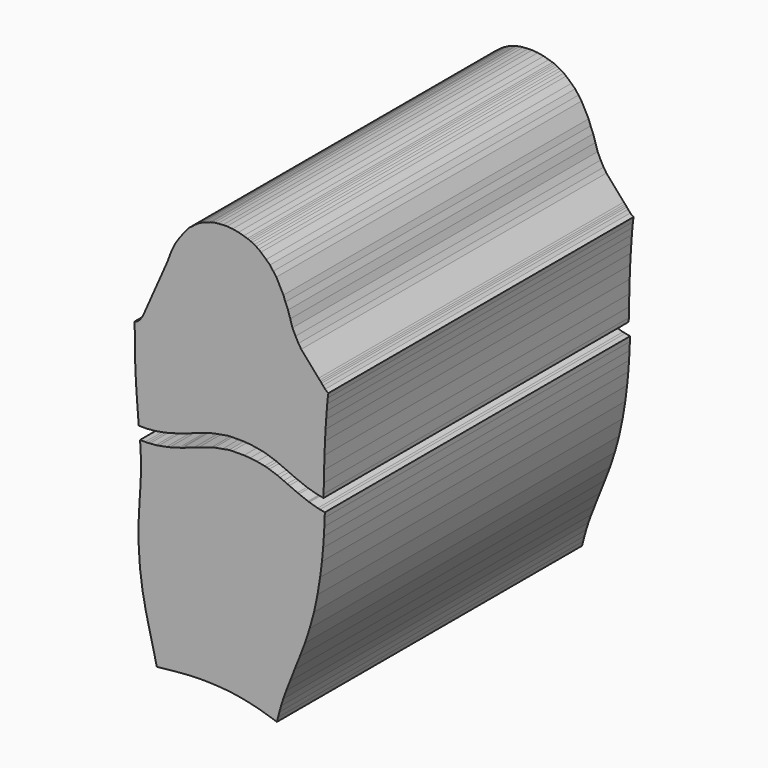
from build123d import *

# Parameters (mm, degrees)
F2_DEPTH = 508


# Not quite as in the source:
# - the program builds the solid bodies; features that only make, move or delete a surface that nothing else refers to are left out


with BuildPart() as f2:
    # F0 (on Front) → F2 (new body)
    with BuildSketch(Plane.XZ):
        Polygon((-99.35524, -267.157394), (-87.704154, -265.912724), (-77.642191, -264.889562), (-67.687226, -263.950115), (-57.626497, -263.202614), (-47.835855, -262.752223), (-37.623644, -262.622648), (-27.549122, -262.832515), (-17.617123, -263.335506), (-7.703785, -264.137581), (1.93555, -265.255393), (11.78373, -266.764753), (21.403733, -268.685028), (30.708282, -270.83535), (39.779716, -273.220339), (47.856634, -275.617817), (54.708213, -277.79442), (60.621898, -279.7178), (62.100178, -273.892381), (63.860292, -267.155842), (66.065188, -259.260817), (68.922512, -250.058256), (72.873976, -239.227413), (78.009644, -226.195026), (84.088358, -210.560021), (90.96442, -193.298534), (97.880029, -175.224811), (104.237719, -155.856182), (109.972263, -134.97015), (114.571321, -113.121317), (118.10686, -91.616372), (120.577504, -72.156973), (122.125705, -55.726912), (123.12777, -41.873435), (123.758995, -30.217446), (124.191324, -19.726469), (124.403661, -13.319637), (118.051474, -12.002012), (114.902297, -11.379006), (103.790009, -8.175114), (102.941473, -7.932579), (102.774185, -7.869009), (101.851989, -7.507658), (90.04621, -2.907224), (87.941009, -2.099751), (77.087624, 2.698767), (74.31532, 3.890768), (69.497222, 5.997663), (64.486402, 8.188801), (61.150429, 9.579169), (50.325408, 13.192707), (47.439086, 14.157448), (44.15215, 14.980091), (33.917572, 16.920968), (24.832063, 18.047035), (16.925466, 18.617653), (1.300727, 18.502788), (-3.02828, 18.408632), (-11.997373, 16.688876), (-22.540419, 14.802432), (-26.847447, 13.566969), (-43.403485, 8.30176), (-49.739938, 6.067019), (-65.069438, 0.721942), (-65.631731, 0.525868), (-66.822744, 0.149595), (-69.900765, -0.691604), (-82.198069, -4.148932), (-86.677218, -5.146552), (-96.860889, -7.030491), (-100.650569, -7.635152), (-108.615022, -8.256464), (-111.81327, -8.50803), (-114.846382, -8.486087), (-121.66787, -8.40389), (-121.242843, -14.793437), (-120.757245, -23.907133), (-120.423058, -34.545006), (-120.480208, -47.140266), (-121.136163, -62.259157), (-122.286607, -80.620535), (-123.449045, -102.956413), (-123.594037, -129.314381), (-121.806265, -157.957926), (-118.219785, -184.666238), (-113.801807, -206.999505), (-109.393073, -225.58084), (-105.540493, -241.278075), (-102.235424, -254.856704), align=None)
    extrude(amount=F2_DEPTH)


with BuildPart() as f2b:
    # F0 (on Front) → F2, piece 2 (new body)
    with BuildSketch(Plane.XZ):
        Polygon((-125.782705, 128.917153), (-129.062374, 127.987089), (-128.75574, 122.909312), (-128.690088, 116.899531), (-128.652305, 109.84454), (-128.59512, 101.393501), (-128.429667, 91.558586), (-128.095552, 79.860298), (-127.522887, 66.053599), (-126.616672, 50.190206), (-125.498014, 34.653661), (-124.489775, 21.756211), (-123.65729, 10.717336), (-123.462027, 7.781413), (-116.640504, 7.699216), (-113.607427, 7.677273), (-110.409179, 7.928839), (-102.444727, 8.550116), (-98.655011, 9.154777), (-88.471375, 11.038751), (-83.992226, 12.036336), (-71.694887, 15.4937), (-68.616865, 16.334898), (-67.425888, 16.711136), (-66.86356, 16.90721), (-51.534095, 22.252322), (-45.197607, 24.487064), (-28.641569, 29.752272), (-24.334541, 30.987735), (-13.79153, 32.874179), (-4.822402, 34.593935), (-0.49343, 34.688092), (15.131344, 34.802921), (23.037906, 34.232338), (32.123415, 33.106271), (42.357992, 31.165394), (45.644929, 30.342716), (48.531251, 29.37801), (59.356307, 25.764472), (62.69228, 24.374104), (67.703065, 22.182931), (72.521198, 20.076036), (75.293502, 18.884035), (86.146851, 14.085552), (88.252088, 13.278079), (100.057832, 8.677645), (100.980063, 8.31626), (101.147315, 8.252689), (101.995852, 8.010154), (113.10814, 4.806262), (116.257317, 4.183291), (122.609539, 2.865631), (122.767831, 7.641643), (123.099548, 20.739082), (123.450808, 36.054012), (123.935843, 53.439183), (124.623971, 70.255465), (125.393379, 84.414377), (126.176334, 96.343487), (126.917803, 106.396948), (127.60639, 114.846011), (128.283264, 121.936033), (129.062374, 127.891945), (124.731004, 131.111007), (121.987627, 134.641254), (120.126725, 136.650077), (118.959418, 138.193339), (117.667546, 139.441255), (116.077118, 141.215586), (92.994833, 167.633279), (89.268511, 173.340024), (85.373809, 180.553236), (81.284021, 188.974853), (78.387857, 198.625724), (75.360777, 207.999347), (71.889514, 216.193034), (69.247244, 223.532964), (59.839825, 241.445503), (55.722414, 247.019109), (51.380707, 252.946199), (46.299402, 257.733958), (39.296269, 263.930641), (36.268519, 266.463621), (32.910886, 268.539683), (30.253622, 269.975876), (27.504425, 271.600524), (25.185158, 272.622098), (23.492248, 273.547928), (21.227027, 274.145851), (16.28267, 275.706081), (9.413205, 277.600145), (1.605491, 279.030694), (-5.790953, 279.717799), (-11.402378, 279.505145), (-17.941749, 279.042724), (-22.593618, 278.590569), (-27.039041, 277.544124), (-30.013804, 276.473549), (-33.890832, 275.292132), (-37.71325, 273.92092), (-40.370866, 272.522579), (-43.719715, 270.766804), (-45.799587, 269.313219), (-48.025791, 267.92465), (-50.056239, 266.236855), (-53.201711, 263.83271), (-56.390082, 261.457457), (-58.186708, 259.497424), (-59.404003, 257.840462), (-61.690532, 255.533648), (-64.17564, 252.118971), (-67.319737, 247.98498), (-71.469497, 242.217945), (-75.866449, 235.03352), (-79.6931, 227.091751), (-82.601188, 219.33385), (-85.060543, 212.654603), (-118.453571, 136.861603), (-119.91975, 134.961824), (-121.672597, 132.711348), (-123.742732, 130.524408), align=None)
    extrude(amount=F2_DEPTH)


solid = Compound([f2.part, f2b.part])
